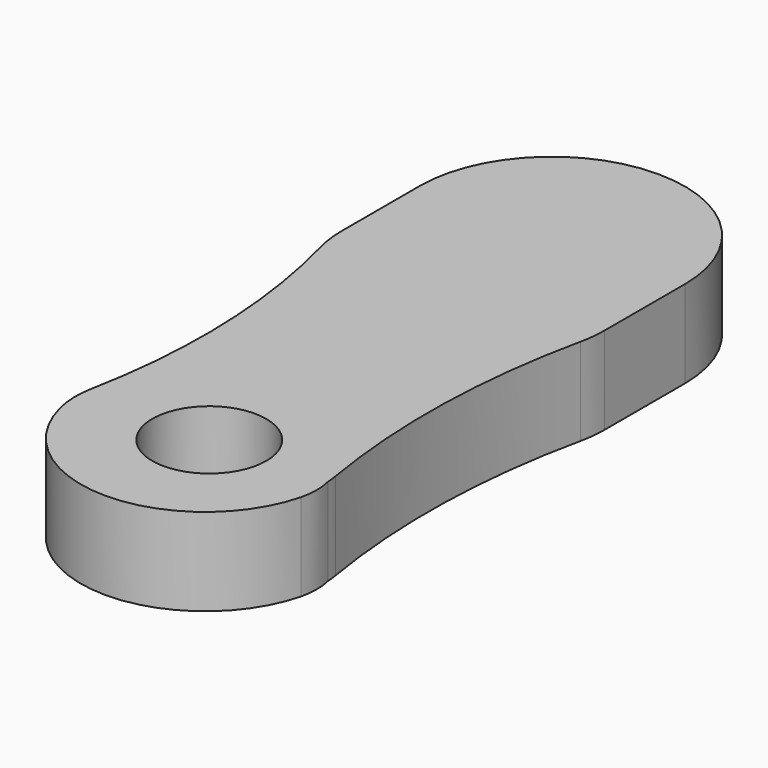
from build123d import *

# Parameters (mm, degrees)
F0_R     = 18.25
F1_DEPTH = 28


# Not quite as in the source:
# - a feature names something its author has since deleted; it is built from what else it names


with BuildPart() as f1:
    # F0 (on Top) → F1 (new body)
    with BuildSketch(Plane.XY):
        with BuildLine():
            Line((23.5539685776, 114.0594776705), (23.1539685776, 114.0594776705))
            ThreePointArc((23.1539685776, 114.0594776705), (-6.7566482666, 101.6700945147), (-19.1460314224, 71.7594776705))
            Line((-19.1460314224, 71.7594776705), (-19.1460314224, 40.5602956202))
            ThreePointArc((-19.1460314224, 40.5602956202), (-18.8100234812, 35.3865412816), (-17.8076447246, 30.2997080702))
            ThreePointArc((-17.8076447246, 30.2997080702), (-10.7929031817, -17.2712382489), (-14.6173474127, -65.2042660996))
            ThreePointArc((-14.6173474127, -65.2042660996), (-15.16027858, -71.7938854137), (-14.2465279536, -78.3423903385))
            ThreePointArc((-14.2465279536, -78.3423903385), (24.3685631197, -108.3214348669), (62.983654193, -78.3423903385))
            ThreePointArc((62.983654193, -78.3423903385), (63.6357145351, -72.9718093248), (62.983654193, -67.6012283111))
            ThreePointArc((62.983654193, -67.6012283111), (62.8457925436, -65.8846278256), (62.6096584736, -64.1787662362))
            ThreePointArc((62.6096584736, -64.1787662362), (59.2183076196, -16.4494096847), (64.932743293, 31.0578314726))
            ThreePointArc((64.932743293, 31.0578314726), (65.6229953988, 35.3006378942), (65.8539685776, 39.593015521))
            Line((65.8539685776, 39.593015521), (65.8539685776, 71.7594776705))
            ThreePointArc((65.8539685776, 71.7594776705), (53.4645854218, 101.6700945147), (23.5539685776, 114.0594776705))
        make_face()
        with Locations((25.6633214675, -68.4624532511)):
            Circle(F0_R, mode=Mode.SUBTRACT)
    extrude(amount=F1_DEPTH)


solid = f1.part
